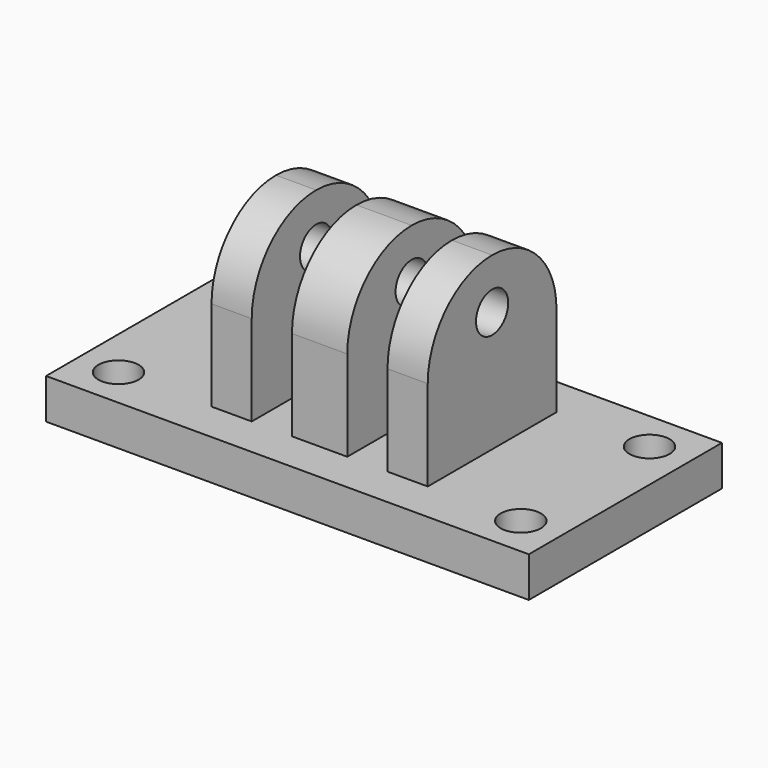
from build123d import *

# Parameters (mm, degrees)
F0_W     = 304.8
F0_H     = 152.4
F0_W_2   = 25.4
F0_H_2   = 101.6
F0_W_3   = 34.925
F1_DEPTH = 25.4
F2_DEPTH = 107.95
F4_DEPTH = 220.6635
F3_R     = 12.7
F5_DEPTH = 220.6635
F6_D     = 25.4


# Not quite as in the source:
# - a feature names something its author has since deleted; it is built from what else it names


with BuildPart() as f1:
    # F0 (on Top) → F1 (new body)
    with BuildSketch(Plane.XY):
        Rectangle(F0_W, F0_H)
        with Locations((-55.5625, 0)):
            Rectangle(F0_W_2, F0_H_2, mode=Mode.SUBTRACT)
        Rectangle(F0_W_3, F0_H_2, mode=Mode.SUBTRACT)
        with Locations((55.5625, 0)):
            Rectangle(F0_W_2, F0_H_2, mode=Mode.SUBTRACT)
        Rectangle(F0_W_3, F0_H_2)
        with Locations((-55.5625, 0)):
            Rectangle(F0_W_2, F0_H_2)
        with Locations((55.5625, 0)):
            Rectangle(F0_W_2, F0_H_2)
    extrude(amount=-F1_DEPTH)

    # F0 (on Top) → F2 (join)
    with BuildSketch(Plane.XY):
        with Locations((55.5625, 0)):
            Rectangle(F0_W_2, F0_H_2)
        Rectangle(F0_W_3, F0_H_2)
        with Locations((-55.5625, 0)):
            Rectangle(F0_W_2, F0_H_2)
    extrude(amount=F2_DEPTH)

    # F3 (on face) → F4 (cut, through all)
    with BuildSketch(Plane.YZ.offset(68.2625)):
        with BuildLine():
            Line((1e-10, 107.95), (-50.8, 107.95))
            Line((-50.8, 107.95), (-50.8, 57.15))
            ThreePointArc((-50.8, 57.15), (-35.9210244842, 93.0710244843), (1e-10, 107.95))
        make_face()
        with BuildLine():
            Line((50.8, 107.95), (1e-10, 107.95))
            ThreePointArc((1e-10, 107.95), (35.9210244843, 93.0710244842), (50.8, 57.15))
            Line((50.8, 57.15), (50.8, 107.95))
        make_face()
    extrude(amount=-F4_DEPTH, mode=Mode.SUBTRACT)

    # F3 (on face) → F5 (cut, through all)
    with BuildSketch(Plane.YZ.offset(68.2625)):
        with Locations((0, 76.2)):
            Circle(F3_R)
    extrude(amount=-F5_DEPTH, mode=Mode.SUBTRACT)

    # F6 (through all)
    with Locations(Plane.XY):
        with Locations((127, -50.8), (127, 50.8), (-127, 50.8), (-127, -50.8)):
            Hole(F6_D / 2)


solid = f1.part
